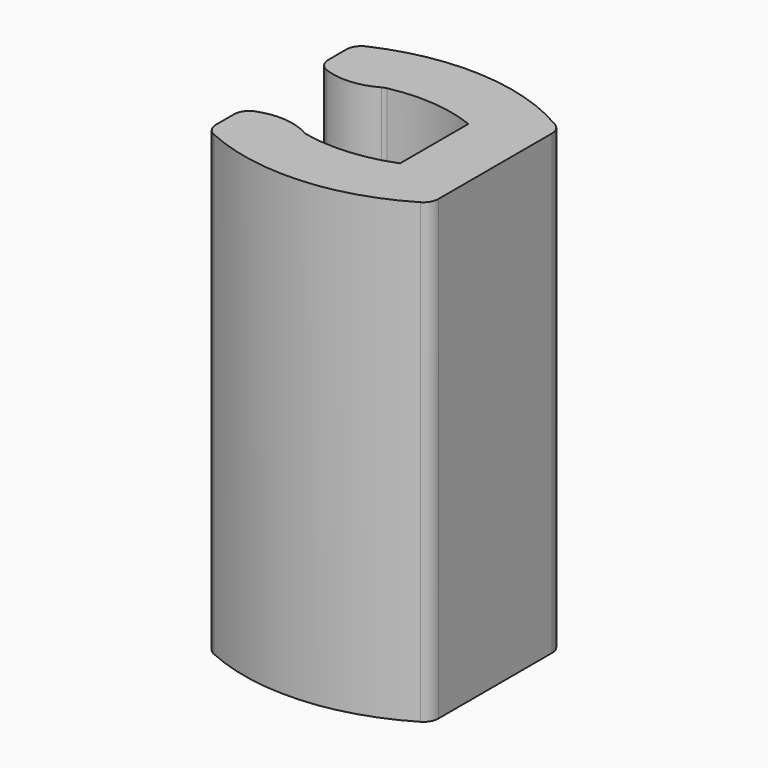
from build123d import *

# Parameters (mm, degrees)
F1_DEPTH = 15
F2_R     = 0.5


with BuildPart() as f1:
    # F0 (on Top) → F1 (new body)
    with BuildSketch(Plane.XY):
        with BuildLine():
            ThreePointArc((0.314997359, 1.625), (1.8064242174, 1.7355083888), (3.2638192562, 1.4))
            Line((3.2638192562, 1.4), (3.2638192562, -1.4))
            ThreePointArc((3.2638192562, -1.4), (1.8064242174, -1.7355083888), (0.314997359, -1.625))
            ThreePointArc((0.314997359, -1.625), (-0.7212203567, -1.3356293712), (-1.7574380725, -1.625))
            Line((-1.7574380725, -1.625), (-1.7574380725, -2.9842268265))
            ThreePointArc((-1.7574380725, -2.9842268265), (1.8043736859, -3.739767503), (5.2638192562, -2.604170276))
            Line((5.2638192562, -2.604170276), (5.2638192562, 2.604170276))
            ThreePointArc((5.2638192562, 2.604170276), (1.8043736859, 3.739767503), (-1.7574380725, 2.9842268265))
            Line((-1.7574380725, 2.9842268265), (-1.7574380725, 1.625))
            ThreePointArc((-1.7574380725, 1.625), (-0.7212203567, 1.3356293712), (0.314997359, 1.625))
        make_face()
    extrude(amount=F1_DEPTH)

    # F2
    f2_edges = [f1.edges().sort_by_distance(p)[0] for p in [
        (0.314997, 1.625, 7.5),
        (0.314997, -1.625, 7.5),
        (-1.757438, -1.625, 7.5),
        (-1.757438, -2.984227, 7.5),
        (5.263819, -2.60417, 7.5),
        (5.263819, 2.60417, 7.5),
        (-1.757438, 2.984227, 7.5),
        (-1.757438, 1.625, 7.5),
    ]]
    fillet(f2_edges, radius=F2_R)


solid = f1.part
